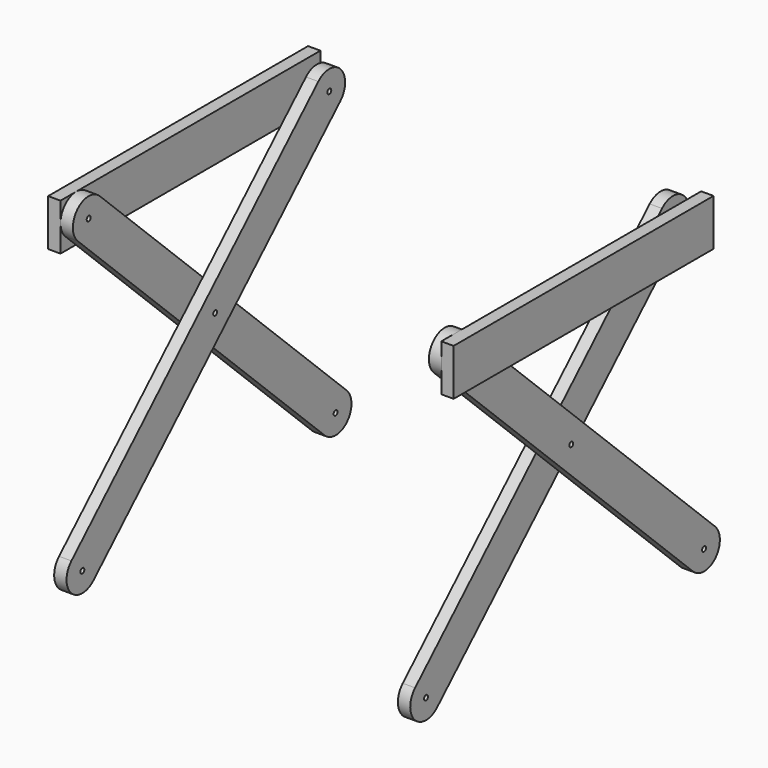
from build123d import *

# Parameters (mm, degrees)
F2_R     = 3.175
F3_DEPTH = 15.875
F4_DEPTH = 15.875
F5_W     = 417.1570104862
F5_H     = 59.898608482
F6_DEPTH = 15.875


# Not quite as in the source:
# - a length typed as a fraction of an inch, garbled in the dataset ("3 / 203.2 mm" for 3/8 in), is restored


with BuildPart() as f3:
    # F2 (on line) → F3 (new body)
    with BuildSketch(Plane.YZ.offset(228.6)):
        with BuildLine():
            Line((36.6633615893, 0), (0, -35.2220263714))
            Line((0, -35.2220263714), (195.5762402522, -223.1096393228))
            ThreePointArc((195.5762402522, -223.1096393228), (231.4900464095, -222.3895509281), (230.7699580147, -186.4757447708))
            Line((230.7699580147, -186.4757447708), (36.6633615893, 0))
        make_face()
        with Locations((213.1730991335, -204.7926920468)):
            Circle(F2_R, mode=Mode.SUBTRACT)
        with BuildLine():
            Line((-200.7753641244, 157.6603189284), (-36.6633615893, 0))
            Line((-36.6633615893, 0), (0, 35.2220263714))
            Line((0, 35.2220263714), (-165.5816463618, 194.2942134805))
            ThreePointArc((-165.5816463618, 194.2942134805), (-201.4954525191, 193.5741250857), (-200.7753641244, 157.6603189284))
        make_face()
        with Locations((-183.1785052431, 175.9772662045)):
            Circle(F2_R, mode=Mode.SUBTRACT)
        Polygon((0, 35.2220263714), (-36.6633615893, 0), (0, -35.2220263714), (36.6633615893, 0), align=None)
        Circle(F2_R, mode=Mode.SUBTRACT)
    extrude(amount=F3_DEPTH)


with BuildPart() as f4:
    # F2 (on line) → F4 (new body)
    with BuildSketch(Plane.YZ.offset(228.6)):
        with BuildLine():
            Line((165.5816463618, 194.2942134805), (0, 35.2220263714))
            Line((0, 35.2220263714), (36.6633615893, 0))
            Line((36.6633615893, 0), (200.7753641244, 157.6603189284))
            ThreePointArc((200.7753641244, 157.6603189284), (201.4954525191, 193.5741250857), (165.5816463618, 194.2942134805))
        make_face()
        with Locations((183.1785052431, 175.9772662045)):
            Circle(F2_R, mode=Mode.SUBTRACT)
        Polygon((0, 35.2220263714), (-36.6633615893, 0), (0, -35.2220263714), (36.6633615893, 0), align=None)
        Circle(F2_R, mode=Mode.SUBTRACT)
        with BuildLine():
            Line((-36.6633615893, 0), (-230.7699580147, -186.4757447708))
            ThreePointArc((-230.7699580147, -186.4757447708), (-231.4900464095, -222.3895509281), (-195.5762402522, -223.1096393228))
            Line((-195.5762402522, -223.1096393228), (0, -35.2220263714))
            Line((0, -35.2220263714), (-36.6633615893, 0))
        make_face()
        with Locations((-213.1730991335, -204.7926920468)):
            Circle(F2_R, mode=Mode.SUBTRACT)
    extrude(amount=-F4_DEPTH)


with BuildPart() as f6:
    # F5 (on face) → F6 (new body)
    with BuildSketch(Plane.YZ.offset(244.475)):
        with Locations((0, 171.4279619635)):
            Rectangle(F5_W, F5_H)
    extrude(amount=F6_DEPTH)


with BuildPart() as f7_1:
    # F7: instance of F4
    add(f4.part.mirror(Plane.YZ))


with BuildPart() as f7_2:
    # F7: instance of F3
    add(f3.part.mirror(Plane.YZ))


with BuildPart() as f7_3:
    # F7: instance of F6
    add(f6.part.mirror(Plane.YZ))


solid = Compound([f3.part, f4.part, f6.part, f7_1.part, f7_2.part, f7_3.part])
